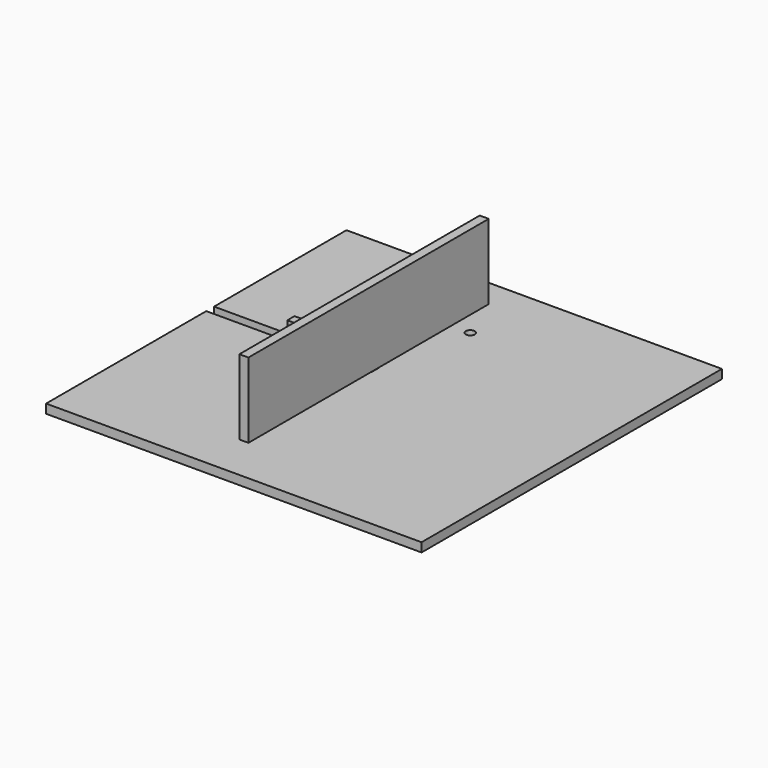
from build123d import *

# Parameters (mm, degrees)
F1_DEPTH  = 12
F3_D      = 12
F4_W      = 12
F4_H      = 400
F5_DEPTH  = 100
F6_W      = 12
F6_H      = 50
F7_DEPTH  = 100
F8_W      = 100
F8_H      = 14
F9_DEPTH  = 25
F10_W     = 100
F10_H     = 13
F11_DEPTH = 25
F12_W     = 100
F12_H     = 12
F13_DEPTH = 25
F14_W     = 45
F14_H     = 91.0748828953
F15_DEPTH = 45


with BuildPart() as f1:
    # F0 (on Top) → F1 (new body)
    with BuildSketch(Plane.XY):
        Polygon((255.0269067287, 249.4558691978), (-244.9730932713, 249.4558691978), (-244.9730932713, 29.0937830806), (-24.9730932713, 29.0937830806), (-24.9730932713, 16.0937830806), (-244.9730932713, 16.0937830806), (-244.9730932713, -250.5441308022), (255.0269067287, -250.5441308022), align=None)
    extrude(amount=F1_DEPTH)

    # F3 (through all)
    with Locations(Plane.XY.offset(12)):
        with Locations((0, 149.4558691978)):
            Hole(F3_D / 2)


with BuildPart() as f5:
    # F4 (on face) → F5 (new body)
    with BuildSketch(Plane.XY.offset(12)):
        with Locations((-31.4178401083, 11.8017673492)):
            Rectangle(F4_W, F4_H)
    extrude(amount=F5_DEPTH)

    # F6 (on face) → F7 (join)
    with BuildSketch(Plane(origin=(-37.4178401083, 0, 0), x_dir=(0, -1, 0), z_dir=(-1, 0, 0))):
        with Locations((-22.5937830806, 11)):
            Rectangle(F6_W, F6_H)
    extrude(amount=F7_DEPTH)

    # F8 (on face) → F9 (join)
    with BuildSketch(Plane.XZ.offset(-16.5937830806)):
        with Locations((-87.4178401083, -7)):
            Rectangle(F8_W, F8_H)
    extrude(amount=F9_DEPTH)

    # F10 (on face) → F11 (join)
    with BuildSketch(Plane(origin=(0, 28.5937830806, 0), x_dir=(-1, 0, 0), z_dir=(0, 1, 0))):
        with Locations((87.4178401083, -7.5)):
            Rectangle(F10_W, F10_H)
    extrude(amount=F11_DEPTH)

    # F12 (on face) → F13 (join)
    with BuildSketch(Plane(origin=(0, 28.5937830806, 0), x_dir=(-1, 0, 0), z_dir=(0, 1, 0))):
        with Locations((87.4178401083, 18)):
            Rectangle(F12_W, F12_H)
    extrude(amount=F13_DEPTH)


with BuildPart() as f15:
    # F14 (on face) → F15 (new body)
    with BuildSketch(Plane(origin=(0, 0, 0), x_dir=(1, 0, 0), z_dir=(0, 0, -1))):
        with Locations((-222.4730932713, -164.2085915056)):
            Rectangle(F14_W, F14_H)
    extrude(amount=F15_DEPTH)


solid = Compound([f1.part, f5.part, f15.part])
